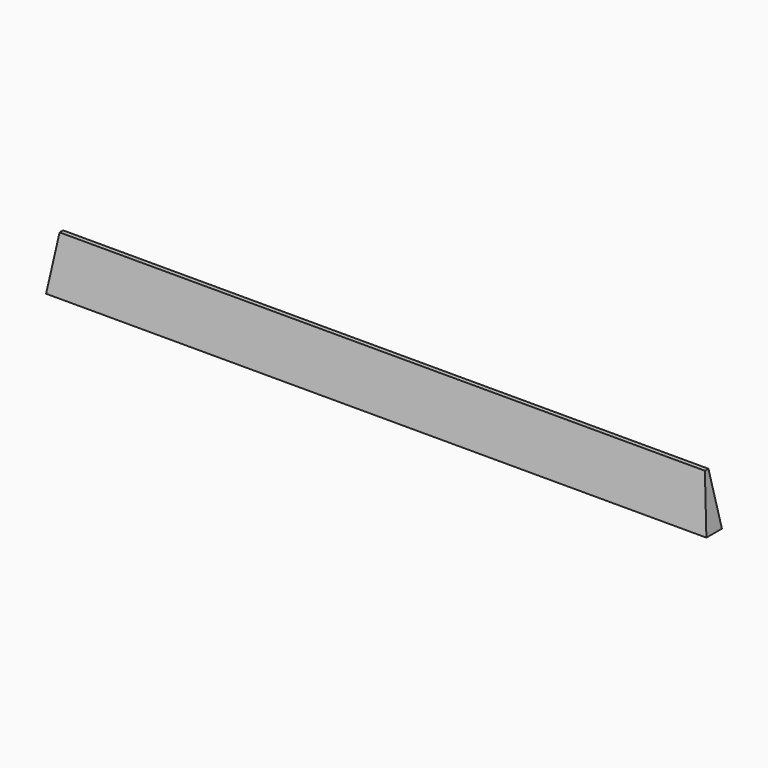
from build123d import *

# Parameters (mm, degrees)
F0_W     = 204
F0_H     = 6
F1_DEPTH = 16.5
F1_TAPER = 8


with BuildPart() as f1:
    # F0 (on Top) → F1 (new body)
    with BuildSketch(Plane.XY):
        with Locations((4.900064, 4.170449)):
            Rectangle(F0_W, F0_H)
    extrude(amount=F1_DEPTH, taper=F1_TAPER)


solid = f1.part
